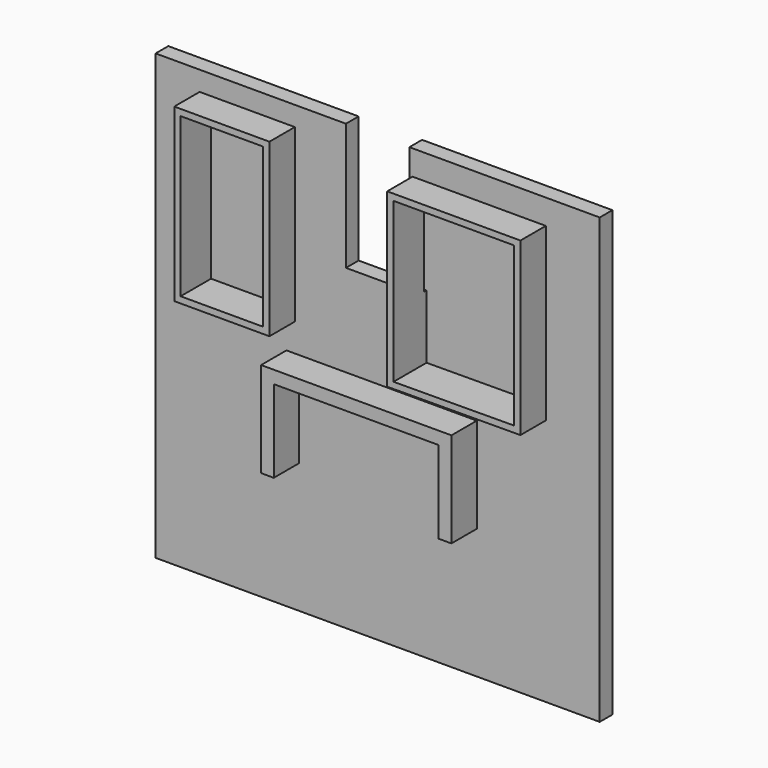
from build123d import *

# Parameters (mm, degrees)
F1_DEPTH = 6.35
F2_W     = 38.1
F2_H     = 68.58
F3_DEPTH = 19.05
F4_T     = -2.54
F6_DEPTH = 19.05
F7_T     = -2.54
F9_DEPTH = 19.05


# Not quite as in the source:
# - a shell that OpenCascade refuses in one call is made with other operations: the cavity is built on its own and cut out


with BuildPart() as f1:
    # F0 (on Front) → F1 (new body)
    with BuildSketch(Plane.XZ):
        Polygon((-90.1848339975, 87.6345549519), (-90.1848339975, -90.1654450481), (87.6151660025, -90.1654450481), (87.6151660025, 87.6345549519), (11.4151660025, 87.6345549519), (11.4151660025, 36.8345549519), (-13.9848339975, 36.8345549519), (-13.9848339975, 87.6345549519), align=None)
    extrude(amount=F1_DEPTH)

    # F2 (on Front) → F3 (join)
    with BuildSketch(Plane.XZ):
        with Locations((-53.5051479423, 45.5094583845)):
            Rectangle(F2_W, F2_H)
    extrude(amount=F3_DEPTH)

    # F4
    f4_openings = [f1.faces().sort_by_distance(p)[0] for p in [
        (-53.505148, -19.05, 45.509458),
    ]]
    offset(amount=F4_T, openings=f4_openings, kind=Kind.INTERSECTION)

    # F5 (on Front) → F6 (join)
    with BuildSketch(Plane.XZ):
        Polygon((12.6932561398, 77.6492066986), (12.6932561398, 8.7867740487), (66.0325084011, 9.0692066986), (66.0325084011, 77.6492066986), align=None)
    extrude(amount=F6_DEPTH)

    # F7: a shell. OpenCascade refuses it in one call, so the cavity is built on its own and cut out:
    # the body offset inwards by the wall thickness, plus a prism from it out through each open face.
    f7_core = offset(f1.part, amount=F7_T, kind=Kind.INTERSECTION, mode=Mode.PRIVATE)
    f7_exits = [f7_core.faces().sort_by_distance(p)[0] for p in [
        (39.346735, -16.51, 43.288574),
    ]]
    add(f7_core, mode=Mode.SUBTRACT)
    extrude(f7_exits, amount=-F7_T, mode=Mode.SUBTRACT)

    # F8 (on Front) → F9 (join)
    with BuildSketch(Plane.XZ):
        Polygon((38.4033048588, 0), (-37.7966951412, 0), (-37.7966951412, -38.1), (-32.7166951412, -38.1), (-32.7166951412, -5.08), (33.3233048588, -5.08), (33.3233048588, -38.1), (38.4033048588, -38.1), align=None)
    extrude(amount=F9_DEPTH)


solid = f1.part
